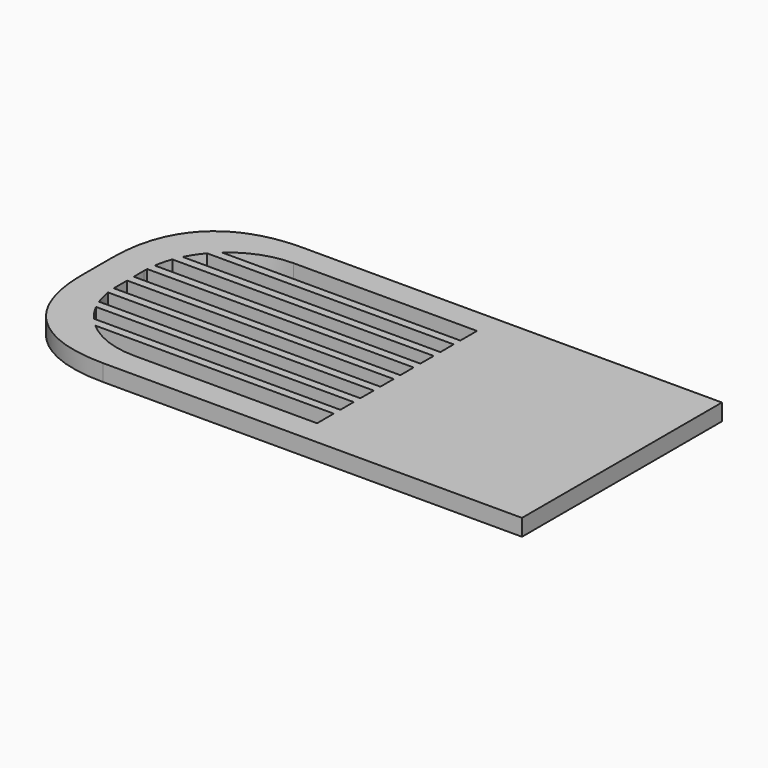
from build123d import *

# Parameters (mm, degrees)
F0_W          = 63
F0_H          = 30
F1_DEPTH      = 2
F2_T1_DEPTH   = 65.5
F3_W          = 32
F3_H          = 24
F4_DEPTH      = 25
F5_R          = 10
F7_E2_W       = 32.4974397272
F7_E2_H       = 2
F7_E3_0_1_0_W = 32.4974397272
F7_E3_0_1_0_H = 2
F7_E3_0_2_0_W = 32.4974397272
F7_E3_0_2_0_H = 2
F7_E3_0_3_0_W = 32.4974397272
F7_E3_0_3_0_H = 2
F7_E3_0_4_0_W = 32.4974397272
F7_E3_0_4_0_H = 2
F7_E3_0_5_0_W = 32.4974397272
F7_E3_0_5_0_H = 2
F7_E3_0_6_0_W = 32.4974397272
F7_E3_0_6_0_H = 2
F8_DEPTH      = 0.5


# Not quite as in the source:
# - a fillet or chamfer that OpenCascade refuses, or shapes differently, is made with other operations: its cross-section is extruded or revolved along the edge and cut away or added


with BuildPart() as f1:
    # F0 (on Top) → F1 (new body)
    with BuildSketch(Plane.XY):
        Rectangle(F0_W, F0_H)
    extrude(amount=F1_DEPTH)

    # F2: fillet of radius 12.7 on 2 edges, made by hand

    # F2_s2 → F2_t1 (cut)
    with BuildSketch(Plane.XY.offset(-31.75)):
        with BuildLine():
            add(Edge.make_bspline(
                [(-18.8, 15), (-31.5, 15), (-31.5, 2.3)],
                knots=[0, 0, 0, 1, 1, 1], degree=2, weights=[1, 0.9230769231, 1]))
            Line((-31.5, 2.3), (-31.5, 15))
            Line((-31.5, 15), (-18.8, 15))
        make_face()
        with BuildLine():
            add(Edge.make_bspline(
                [(-31.5, -2.3), (-31.5, -15), (-18.8, -15)],
                knots=[0, 0, 0, 1, 1, 1], degree=2, weights=[1, 0.9230769231, 1]))
            Line((-18.8, -15), (-31.5, -15))
            Line((-31.5, -15), (-31.5, -2.3))
        make_face()
    extrude(amount=F2_T1_DEPTH, mode=Mode.SUBTRACT)

    # F3 (on face) → F4 (cut)
    with BuildSketch(Plane.XY.offset(2)):
        with Locations((-11.5, 0)):
            Rectangle(F3_W, F3_H)
    extrude(amount=-F4_DEPTH, mode=Mode.SUBTRACT)

    # F5
    f5_edges = [f1.edges().sort_by_distance(p)[0] for p in [
        (-27.5, 12, 1),
        (-27.5, -12, 1),
    ]]
    fillet(f5_edges, radius=F5_R)

    # F7_E2 (on explicit) + F7_E3_0_1_0 (on explicit) + F7_E3_0_2_0 (on explicit) + F7_E3_0_3_0 (on explicit) + F7_E3_0_4_0 (on explicit) + F7_E3_0_5_0 (on explicit) + F7_E3_0_6_0 (on explicit) → F8 (join, symmetric)
    with BuildSketch(Plane(origin=(4.5, -9, 2), x_dir=(-1, 0, 0), z_dir=(0, -1, 0))):
        with Locations((16.2487198636, 1)):
            Rectangle(F7_E2_W, F7_E2_H)
    with BuildSketch(Plane(origin=(4.5, -6, 2), x_dir=(-1, 0, 0), z_dir=(0, -1, 0))):
        with Locations((16.2487198636, 1)):
            Rectangle(F7_E3_0_1_0_W, F7_E3_0_1_0_H)
    with BuildSketch(Plane(origin=(4.5, -3, 2), x_dir=(-1, 0, 0), z_dir=(0, -1, 0))):
        with Locations((16.2487198636, 1)):
            Rectangle(F7_E3_0_2_0_W, F7_E3_0_2_0_H)
    with BuildSketch(Plane(origin=(4.5, 0, 2), x_dir=(-1, 0, 0), z_dir=(0, -1, 0))):
        with Locations((16.2487198636, 1)):
            Rectangle(F7_E3_0_3_0_W, F7_E3_0_3_0_H)
    with BuildSketch(Plane(origin=(4.5, 3, 2), x_dir=(-1, 0, 0), z_dir=(0, -1, 0))):
        with Locations((16.2487198636, 1)):
            Rectangle(F7_E3_0_4_0_W, F7_E3_0_4_0_H)
    with BuildSketch(Plane(origin=(4.5, 6, 2), x_dir=(-1, 0, 0), z_dir=(0, -1, 0))):
        with Locations((16.2487198636, 1)):
            Rectangle(F7_E3_0_5_0_W, F7_E3_0_5_0_H)
    with BuildSketch(Plane(origin=(4.5, 9, 2), x_dir=(-1, 0, 0), z_dir=(0, -1, 0))):
        with Locations((16.2487198636, 1)):
            Rectangle(F7_E3_0_6_0_W, F7_E3_0_6_0_H)
    extrude(amount=F8_DEPTH, both=True)


solid = f1.part
